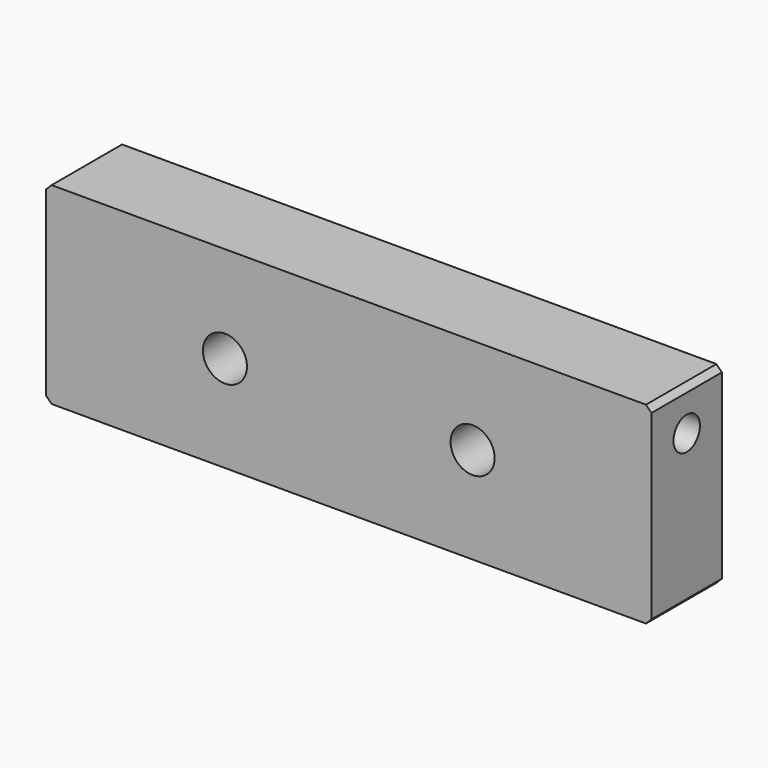
from build123d import *

# Parameters (mm, degrees)
F1_W     = 10
F1_H     = 35.0110880776
F1_W_2   = 90
F1_R     = 5
F2_DEPTH = 16
F3_SIZE  = 1
F7_DEPTH = 12


# Not quite as in the source:
# - a feature of the source that left no trace in its solid (it failed there, or was rolled back) is left out
# - a pattern or mirror of a feature is missing from the dataset's text; its kind, count and spacing are read off the source's solid


with BuildPart() as f2:
    # F1 (on Front) → F2 (new body)
    with BuildSketch(Plane.XZ):
        with Locations((-50, 0)):
            Rectangle(F1_W, F1_H)
        Rectangle(F1_W_2, F1_H)
        with Locations((-35, 0)):
            Circle(F1_R, mode=Mode.SUBTRACT)
        with BuildLine():
            ThreePointArc((-26.5, 0), (-22.5, 4), (-18.5, 0))
            ThreePointArc((-18.5, 0), (-22.5, -4), (-26.5, 0))
        make_face(mode=Mode.SUBTRACT)
        with BuildLine():
            ThreePointArc((26.5, 0), (22.5, -4), (18.5, 0))
            ThreePointArc((18.5, 0), (22.5, 4), (26.5, 0))
        make_face(mode=Mode.SUBTRACT)
        with BuildLine():
            ThreePointArc((40, 0), (35, -5), (30, 0))
            ThreePointArc((30, 0), (35, 5), (40, 0))
        make_face(mode=Mode.SUBTRACT)
        with Locations((-35, 0)):
            Circle(F1_R)
        with BuildLine():
            ThreePointArc((40, 0), (35, 5), (30, 0))
            ThreePointArc((30, 0), (35, -5), (40, 0))
        make_face()
        with Locations((50, 0)):
            Rectangle(F1_W, F1_H)
    extrude(amount=-F2_DEPTH)

    # F3
    f3_edges = [f2.edges().sort_by_distance(p)[0] for p in [
        (55, 8, -17.505544),
        (55, 8, 17.505544),
        (-55, 8, -17.505544),
        (-55, 8, 17.505544),
    ]]
    chamfer(f3_edges, length=F3_SIZE)

    # F4 (on offset) → F5 (revolve, cut)
    with BuildSketch(Plane.XY.offset(10)):
        Polygon((57.6581534887, 5), (57.6581534887, 8), (-50, 8), (-48.1974181429, 5), align=None)
    revolve(axis=Axis((3.8290767443, 8, 10), (-1, 0, 0)), mode=Mode.SUBTRACT)

    # F6 (on face) → F7 (cut)
    with BuildSketch(Plane(origin=(0, 16, 0), x_dir=(-1, 0, 0), z_dir=(0, 1, 0))):
        with BuildLine():
            Line((30, 6), (30, 0))
            ThreePointArc((30, 0), (35, -5), (40, 0))
            Line((40, 0), (40, 6))
            ThreePointArc((40, 6), (35, 11), (30, 6))
        make_face()
    f7 = extrude(amount=-F7_DEPTH, mode=Mode.SUBTRACT)

    # F7_copies: F7 across plane
    add(f7.mirror(Plane(origin=(0, 0, 0), x_dir=(0, 0, 1), z_dir=(1, 0, 0))), mode=Mode.SUBTRACT)


solid = f2.part
